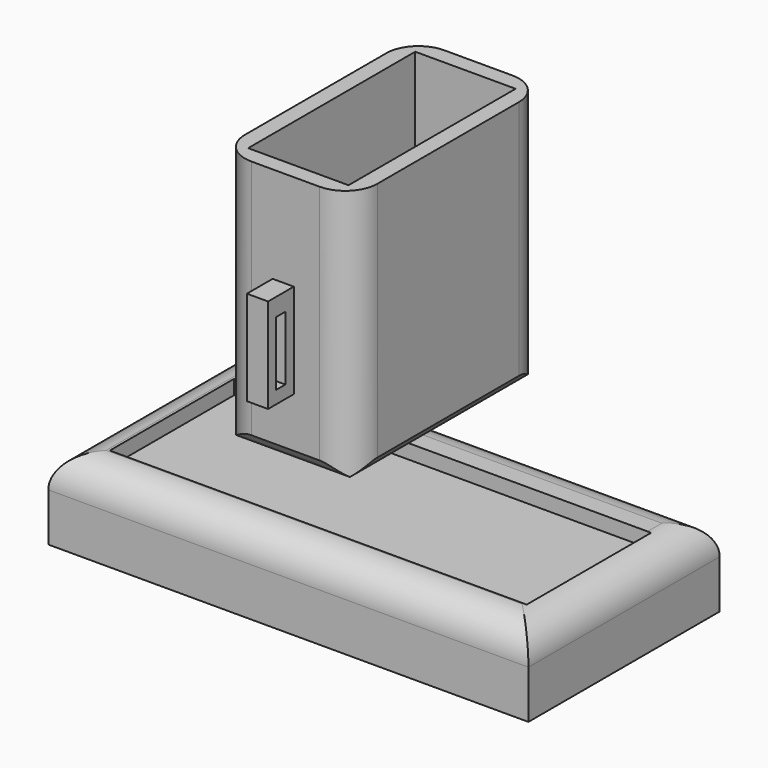
from build123d import *

# Parameters (mm, degrees)
F0_W         = 75.910821557
F0_H         = 37.8035865724
F1_DEPTH     = 12.7
F2_W         = 65.8906013705
F2_H         = 24.5951046236
F3_DEPTH     = 2.286
F7_T1_DEPTH  = 101.310821557
F7_T3_DEPTH  = 63.2035865724
F8_W         = 20.9513884038
F8_H         = 2.7327910066
F9_DEPTH     = 38.1
F10_T1_DEPTH = 43.477489898
F10_T3_DEPTH = 60.6261014942
F11_W        = 20.9513884038
F11_H        = 38.1
F12_DEPTH    = 38.1
F13_T        = -2.54
F14_R        = 5.08
F15_R        = 5.08
F16_W        = 3.3429935575
F16_H        = 14.9679705501
F17_DEPTH    = 5.08
F18_W        = 1.8081573071
F18_H        = 10.1374536753
F19_DEPTH    = 5.08
F20_W        = 3.0222646892
F20_H        = 12.5214233994
F21_DEPTH    = 5.08
F22_W        = 1.8191151321
F22_H        = 8.0005712807
F23_DEPTH    = 5.08


# Not quite as in the source:
# - a fillet or chamfer that OpenCascade refuses, or shapes differently, is made with other operations: its cross-section is extruded or revolved along the edge and cut away or added
# - the program builds the solid bodies; features that only make, move or delete a surface that nothing else refers to are left out


with BuildPart() as f1:
    # F0 (on Top) → F1 (new body)
    with BuildSketch(Plane.XY):
        with Locations((37.9554107785, 18.9017932862)):
            Rectangle(F0_W, F0_H)
    extrude(amount=F1_DEPTH)

    # F2 (on face) → F3 (cut)
    with BuildSketch(Plane.XY.offset(12.7)):
        with Locations((38.4108766448, 17.6113096531)):
            Rectangle(F2_W, F2_H)
    extrude(amount=-F3_DEPTH, mode=Mode.SUBTRACT)

    # F7: fillet of radius 5.08 on 4 edges, made by hand

    # F7_s2 → F7_t1 (cut)
    with BuildSketch(Plane.YZ.offset(-12.7)):
        with BuildLine():
            ThreePointArc((0, 7.62), (1.4878975516, 11.2121024484), (5.08, 12.7))
            Line((5.08, 12.7), (0, 12.7))
            Line((0, 12.7), (0, 7.62))
        make_face()
        with BuildLine():
            ThreePointArc((37.8035865724, 7.62), (36.3156890208, 11.2121024484), (32.7235865724, 12.7))
            Line((32.7235865724, 12.7), (37.8035865724, 12.7))
            Line((37.8035865724, 12.7), (37.8035865724, 7.62))
        make_face()
    extrude(amount=F7_T1_DEPTH, mode=Mode.SUBTRACT)

    # F7_s4 → F7_t3 (cut)
    with BuildSketch(Plane.XZ.offset(-50.5035865724)):
        with BuildLine():
            ThreePointArc((0, 7.62), (1.4878975516, 11.2121024484), (5.08, 12.7))
            Line((5.08, 12.7), (0, 12.7))
            Line((0, 12.7), (0, 7.62))
        make_face()
        with BuildLine():
            ThreePointArc((70.830821557, 12.7), (74.4229240055, 11.2121024484), (75.910821557, 7.62))
            Line((75.910821557, 7.62), (75.910821557, 12.7))
            Line((75.910821557, 12.7), (70.830821557, 12.7))
        make_face()
    extrude(amount=F7_T3_DEPTH, mode=Mode.SUBTRACT)


with BuildPart() as f9:
    # F8 (on Front) → F9 (new body)
    with BuildSketch(Plane.XZ):
        with Locations((37.4999428168, 24.2914613336)):
            Rectangle(F8_W, F8_H)
    extrude(amount=-F9_DEPTH)

    # F10: fillet of radius 5.08 on 4 edges, made by hand

    # F10_s2 → F10_t1 (cut)
    with BuildSketch(Plane.YZ.offset(15.7611978678)):
        with BuildLine():
            ThreePointArc((4.5052202988, 22.9250658303), (1.8705876572, 23.6616672943), (0, 25.6578568369))
            Line((0, 25.6578568369), (0, 22.9250658303))
            Line((0, 22.9250658303), (4.5052202988, 22.9250658303))
        make_face()
        with BuildLine():
            ThreePointArc((33.5947797012, 22.9250658303), (36.2294123428, 23.6616672943), (38.1, 25.6578568369))
            Line((38.1, 25.6578568369), (38.1, 22.9250658303))
            Line((38.1, 22.9250658303), (33.5947797012, 22.9250658303))
        make_face()
    extrude(amount=F10_T1_DEPTH, mode=Mode.SUBTRACT)

    # F10_s4 → F10_t3 (cut)
    with BuildSketch(Plane.XZ.offset(-49.3630507471)):
        with BuildLine():
            ThreePointArc((43.4704167198, 22.9250658303), (46.1050493615, 23.6616672943), (47.9756370187, 25.6578568369))
            Line((47.9756370187, 25.6578568369), (47.9756370187, 22.9250658303))
            Line((47.9756370187, 22.9250658303), (43.4704167198, 22.9250658303))
        make_face()
        with BuildLine():
            ThreePointArc((27.0242486149, 25.6578568369), (28.8948362721, 23.6616672943), (31.5294689138, 22.9250658303))
            Line((31.5294689138, 22.9250658303), (27.0242486149, 22.9250658303))
            Line((27.0242486149, 22.9250658303), (27.0242486149, 25.6578568369))
        make_face()
    extrude(amount=F10_T3_DEPTH, mode=Mode.SUBTRACT)

    # F11 (on face) → F12 (join)
    with BuildSketch(Plane.XY.offset(25.6578568369)):
        with Locations((37.4999428168, 19.05)):
            Rectangle(F11_W, F11_H)
    extrude(amount=F12_DEPTH)

    # F13
    f13_openings = [f9.faces().sort_by_distance(p)[0] for p in [
        (37.499943, 19.05, 63.757857),
    ]]
    offset(amount=F13_T, openings=f13_openings)

    # F14
    f14_edges = [f9.edges().sort_by_distance(p)[0] for p in [
        (47.975637, 38.1, 44.707857),
        (47.975637, 0, 44.707857),
        (27.024249, 38.1, 44.707857),
    ]]
    fillet(f14_edges, radius=F14_R)

    # F15
    f15_edges = [f9.edges().sort_by_distance(p)[0] for p in [
        (27.024249, 0, 44.707857),
    ]]
    fillet(f15_edges, radius=F15_R)

    # F16 (on face) → F17 (join)
    with BuildSketch(Plane.XZ):
        with Locations((37.1399968863, 41.0371609032)):
            Rectangle(F16_W, F16_H)
    extrude(amount=F17_DEPTH)

    # F18 (on face) → F19 (cut)
    with BuildSketch(Plane(origin=(35.4685001075, 0, 0), x_dir=(0, -1, 0), z_dir=(-1, 0, 0))):
        with Locations((2.5656485814, 40.6363867223)):
            Rectangle(F18_W, F18_H)
    extrude(amount=-F19_DEPTH, mode=Mode.SUBTRACT)

    # F20 (on face) → F21 (join)
    with BuildSketch(Plane(origin=(0, 38.1, 0), x_dir=(-1, 0, 0), z_dir=(0, 1, 0))):
        with Locations((-37.3821165413, 38.5855287313)):
            Rectangle(F20_W, F20_H)
    extrude(amount=F21_DEPTH)

    # F22 (on face) → F23 (cut)
    with BuildSketch(Plane.YZ.offset(38.8932488859)):
        with Locations((40.9287344664, 38.0991082639)):
            Rectangle(F22_W, F22_H)
    extrude(amount=-F23_DEPTH, mode=Mode.SUBTRACT)


solid = Compound([f1.part, f9.part])
